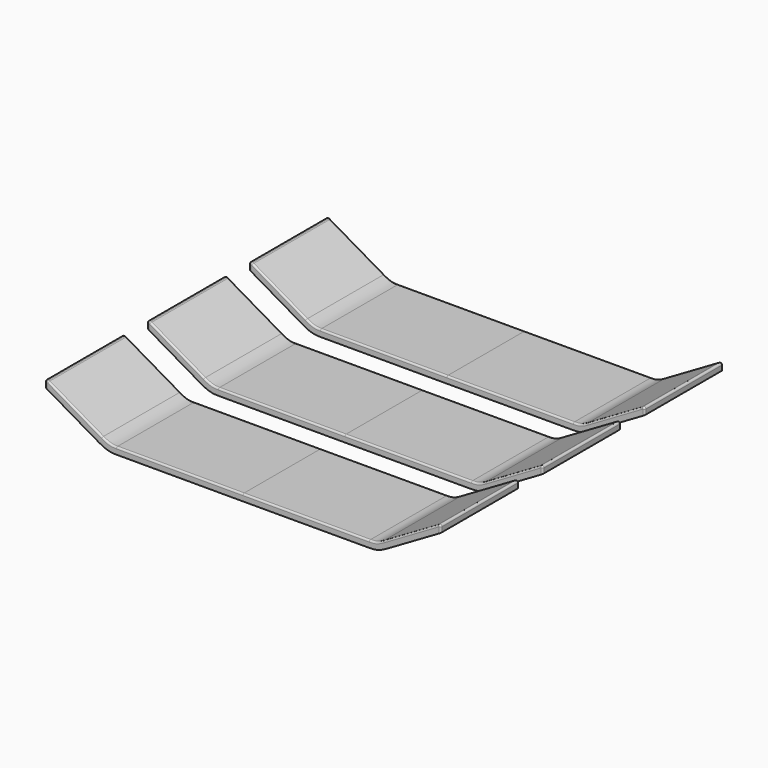
from build123d import *

# Parameters (mm, degrees)
F1_DEPTH = 146.05
F2_R     = 2.54


with BuildPart() as f1:
    # F0 (on Front) → F1 (new body)
    with BuildSketch(Plane.XZ):
        with BuildLine():
            Line((1.5943159571, 65.9026825806), (1.5943159571, 54.15516499))
            Line((1.5943159571, 54.15516499), (81.9025710225, 7.5405244716))
            add(Edge.make_bspline(
                [(81.9025710225, 7.5405244716), (92.2999233007, 1.5054497635), (98.6241698265, 0), (108.1725358963, 0)],
                knots=[0, 0, 0, 0, 27.3307622246, 27.3307622246, 27.3307622246, 27.3307622246], degree=3))
            Line((108.1725358963, 0), (113.0361670146, -2.841e-07))
            Line((113.0361670146, -2.841e-07), (138.4361670146, -1.768e-06))
            Line((138.4361670146, -1.768e-06), (297.1861670146, -1.10422e-05))
            Line((297.1861670146, -1.10422e-05), (297.1800001915, 10.1599889582))
            Line((297.1800001915, 10.1599889582), (108.1725311829, 10.16))
            add(Edge.make_bspline(
                [(87.0029645505, 16.3275368114), (88.1885538875, 15.6393696743), (90.3942484594, 14.4210715514), (93.2713691382, 13.0231304302), (95.7978416249, 11.994384017), (98.0869107324, 11.2602812726), (100.2922847586, 10.7469020057), (102.5915460742, 10.4019914085), (105.1499671195, 10.2020688941), (107.1124775165, 10.1600000624), (108.1725311829, 10.16)],
                knots=[7.897e-07, 7.897e-07, 7.897e-07, 7.897e-07, 0.125, 0.25, 0.375, 0.5, 0.625, 0.75, 0.875, 0.9999998147, 0.9999998147, 0.9999998147, 0.9999998147], degree=3))
            Line((87.0029645505, 16.3275368113), (6.6947068499, 62.9421788594))
            Line((6.6947068499, 62.9421788594), (1.5943159571, 65.9026825806))
        make_face()
    extrude(amount=F1_DEPTH)

    # F2
    f2_edges = [f1.edges().sort_by_distance(p)[0] for p in [
        (202.676266, 0, 10.159994),
        (97.116174, 0, 11.580578),
        (44.29864, 0, 41.11511),
        (1.594316, -73.025, 65.902683),
        (44.29864, -146.05, 41.11511),
        (97.116174, -146.05, 11.580578),
        (202.676266, -146.05, 10.159994),
        (1.594316, -146.05, 60.028924),
        (1.594316, 0, 60.028924),
    ]]
    fillet(f2_edges, radius=F2_R)

    # F3: F1 across face


with BuildPart() as f1_1:
    add(f1.part)
    add(f1.part.mirror(Plane(origin=(297.1830887239, -73.025, 5.0715521532), x_dir=(0, 1, 0), z_dir=(0.9999998158, 0, 0.0006069707))))


with BuildPart() as f4_1:
    # F4: copy of F1
    add(f1_1.part.moved(Location((0, 190.5, 0))))


with BuildPart() as f5_1:
    # F5: copy of F4_1
    add(f4_1.part.moved(Location((0, 190.5, 0))))


solid = Compound([f1_1.part, f4_1.part, f5_1.part])
